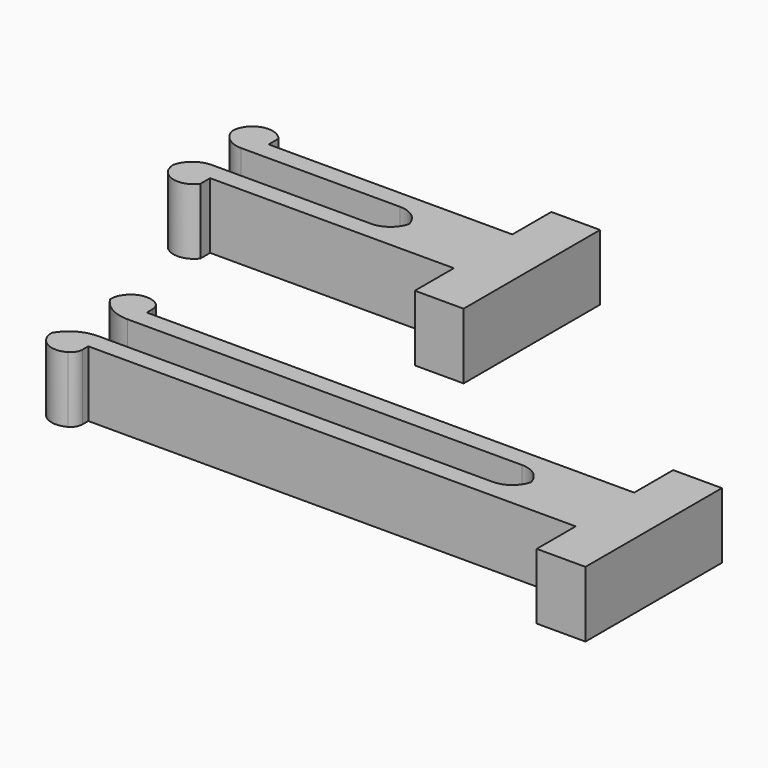
from build123d import *

# Parameters (mm, degrees)
F1_DEPTH    = 2.7
F2_R        = 0.5
F3_T1_DEPTH = 9.1951905284
F4_T1_DEPTH = 2.7
F7_DEPTH    = 2.7
F8_T1_DEPTH = 7.5412291828
F9_T1_DEPTH = 2.7


# Not quite as in the source:
# - a fillet or chamfer that OpenCascade refuses, or shapes differently, is made with other operations: its cross-section is extruded or revolved along the edge and cut away or added


with BuildPart() as f1:
    # F0 (on Top) → F1 (new body)
    with BuildSketch(Plane.XY):
        Polygon((10.75, -1.5), (10.75, 1.5), (-9.25, 1.5), (-10.75, 1.5), (-10.75, 0.75), (7.75, 0.75), (7.75, -0.75), (-10.75, -0.75), (-10.75, -1.5), (-9.25, -1.5), align=None)
        Polygon((10.75, 3.5), (10.75, 1.5), (10.75, -1.5), (10.75, -3.5), (12.75, -3.5), (12.75, 3.5), align=None)
        with BuildLine():
            Line((-10.75, 1.5), (-9.25, 1.5))
            Line((-9.25, 1.5), (-9.25, 2))
            ThreePointArc((-9.25, 2), (-10.180189805, 2.290569415), (-10.75, 1.5))
        make_face()
        with BuildLine():
            Line((-9.25, -2), (-9.25, -1.5))
            Line((-9.25, -1.5), (-10.75, -1.5))
            ThreePointArc((-10.75, -1.5), (-10.180189805, -2.290569415), (-9.25, -2))
        make_face()
    extrude(amount=F1_DEPTH)

    # F2
    f2_edges = [f1.edges().sort_by_distance(p)[0] for p in [
        (-9.25, 2, 1.35),
        (-9.25, -2, 1.35),
    ]]
    fillet(f2_edges, radius=F2_R)

    # F3: fillet of radius 1.5 on 2 edges, made by hand

    # F3_s2 → F3_t1 (cut)
    with BuildSketch(Plane.XY.offset(-3.2475952642)):
        with BuildLine():
            ThreePointArc((-10.75, 1.5), (-10.2009618943, 0.9509618943), (-9.4509618943, 0.75))
            Line((-9.4509618943, 0.75), (-10.75, 0.75))
            Line((-10.75, 0.75), (-10.75, 1.5))
        make_face()
        with BuildLine():
            ThreePointArc((-9.4509618943, -0.75), (-10.2009618943, -0.9509618943), (-10.75, -1.5))
            Line((-10.75, -1.5), (-10.75, -0.75))
            Line((-10.75, -0.75), (-9.4509618943, -0.75))
        make_face()
    extrude(amount=F3_T1_DEPTH, mode=Mode.SUBTRACT)

    # F4: fillet of radius 1 on 2 edges, made by hand

    # F4_s2 → F4_t1 (join)
    with BuildSketch(Plane.XY):
        with BuildLine():
            ThreePointArc((7.75, -0.25), (7.4571067812, 0.4571067812), (6.75, 0.75))
            Line((6.75, 0.75), (7.75, 0.75))
            Line((7.75, 0.75), (7.75, -0.25))
        make_face()
        with BuildLine():
            ThreePointArc((6.75, -0.75), (7.4571067812, -0.4571067812), (7.75, 0.25))
            Line((7.75, 0.25), (7.75, -0.75))
            Line((7.75, -0.75), (6.75, -0.75))
        make_face()
    extrude(amount=F4_T1_DEPTH)


with BuildPart() as f7:
    # F6 (on offset) → F7 (new body)
    with BuildSketch(Plane.XY.offset(7.7)):
        Polygon((5.75, 3.5), (5.75, 1.5), (5.75, -1.5), (5.75, -3.5), (7.75, -3.5), (7.75, 3.5), align=None)
        Polygon((5.75, -1.5), (5.75, 1.5), (-4.25, 1.5), (-5.75, 1.5), (-5.75, 0.75), (2.75, 0.75), (2.75, -0.75), (-5.75, -0.75), (-5.75, -1.5), (-4.25, -1.5), align=None)
        with BuildLine():
            Line((-5.75, 1.5), (-4.25, 1.5))
            Line((-4.25, 1.5), (-4.25, 2))
            ThreePointArc((-4.25, 2), (-5.180189805, 2.290569415), (-5.75, 1.5))
        make_face()
        with BuildLine():
            Line((-4.25, -2), (-4.25, -1.5))
            Line((-4.25, -1.5), (-5.75, -1.5))
            ThreePointArc((-5.75, -1.5), (-5.180189805, -2.290569415), (-4.25, -2))
        make_face()
    extrude(amount=F7_DEPTH)

    # F8: fillet of radius 1 on 2 edges, made by hand

    # F8_s2 → F8_t1 (cut)
    with BuildSketch(Plane.XY.offset(5.2793854086)):
        with BuildLine():
            ThreePointArc((-5.75, 1.5), (-5.3941265991, 0.959430585), (-4.7817541634, 0.75))
            Line((-4.7817541634, 0.75), (-5.75, 0.75))
            Line((-5.75, 0.75), (-5.75, 1.5))
        make_face()
        with BuildLine():
            ThreePointArc((-4.7817541634, -0.75), (-5.3941265991, -0.959430585), (-5.75, -1.5))
            Line((-5.75, -1.5), (-5.75, -0.75))
            Line((-5.75, -0.75), (-4.7817541634, -0.75))
        make_face()
    extrude(amount=F8_T1_DEPTH, mode=Mode.SUBTRACT)

    # F9: fillet of radius 1 on 2 edges, made by hand

    # F9_s2 → F9_t1 (join)
    with BuildSketch(Plane.XY.offset(7.7)):
        with BuildLine():
            ThreePointArc((2.75, -0.25), (2.4571067812, 0.4571067812), (1.75, 0.75))
            Line((1.75, 0.75), (2.75, 0.75))
            Line((2.75, 0.75), (2.75, -0.25))
        make_face()
        with BuildLine():
            ThreePointArc((1.75, -0.75), (2.4571067812, -0.4571067812), (2.75, 0.25))
            Line((2.75, 0.25), (2.75, -0.75))
            Line((2.75, -0.75), (1.75, -0.75))
        make_face()
    extrude(amount=F9_T1_DEPTH)


solid = Compound([f1.part, f7.part])
